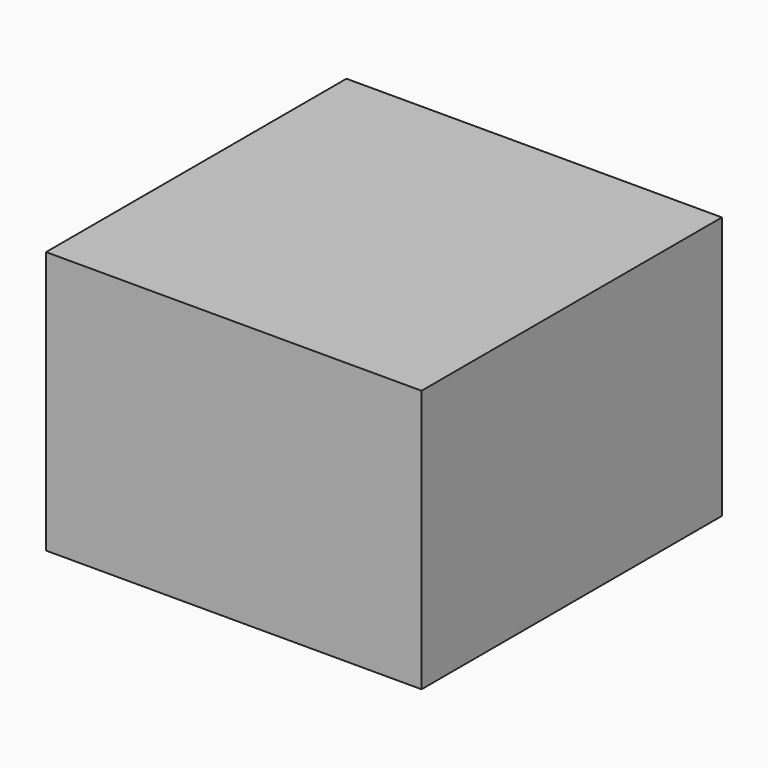
from build123d import *

# Parameters (mm, degrees)
F0_W     = 100
F0_H     = 100
F3_DEPTH = 70


# Not quite as in the source:
# - a feature of the source that left no trace in its solid (it failed there, or was rolled back) is left out


with BuildPart() as f3:
    # F0 (on Top) → F3 (new body)
    with BuildSketch(Plane.XY):
        Rectangle(F0_W, F0_H)
    extrude(amount=F3_DEPTH)


solid = f3.part
